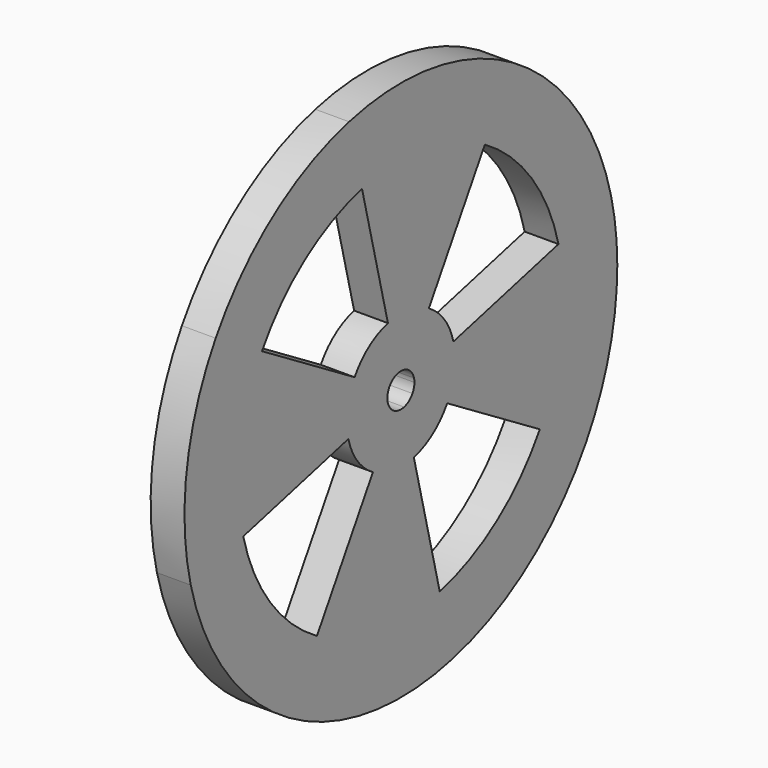
from build123d import *

# Parameters (mm, degrees)
F1_DEPTH = 3.175


with BuildPart() as f1:
    # F0 (on Right) → F1 (new body)
    with BuildSketch(Plane.YZ):
        with BuildLine():
            Line((-40.4511333859, 29.1073653109), (-36.3753204967, 26.6437996954))
            ThreePointArc((-36.3753204967, 26.6437996954), (-35.6929146046, 28.2235683845), (-35.4597376823, 29.9285538495))
            ThreePointArc((-35.4597376823, 29.9285538495), (-35.506060347, 30.6941595257), (-35.6443525017, 31.4485951564))
            Line((-35.6443525017, 31.4485951564), (-40.2683913872, 30.3085641762))
            ThreePointArc((-40.2683913872, 30.3085641762), (-40.2338183485, 30.1199552685), (-40.2222376823, 29.9285538495))
            ThreePointArc((-40.2222376823, 29.9285538495), (-40.2805319129, 29.5023074832), (-40.4511333859, 29.1073653109))
        make_face()
        with BuildLine():
            ThreePointArc((-40.2896963754, 23.7631686688), (-38.0460118676, 24.8141752957), (-36.3753204967, 26.6437996954))
            Line((-36.3753204967, 26.6437996954), (-40.4511333859, 29.1073653109))
            ThreePointArc((-40.4511333859, 29.1073653109), (-40.8688062286, 28.649959211), (-41.4297273556, 28.3872075543))
            Line((-41.4297273556, 28.3872075543), (-40.2896963754, 23.7631686688))
        make_face()
        with BuildLine():
            ThreePointArc((-35.4597376823, 29.9285538495), (-35.6929146046, 28.2235683845), (-36.3753204967, 26.6437996954))
            Line((-36.3753204967, 26.6437996954), (-25.5064861254, 20.0742913873))
            ThreePointArc((-25.5064861254, 20.0742913873), (-23.4592684491, 24.8135974547), (-22.7597376823, 29.9285538495))
            ThreePointArc((-22.7597376823, 29.9285538495), (-22.8987056762, 32.2253708783), (-23.3135821405, 34.4886777702))
            Line((-23.3135821405, 34.4886777702), (-35.6443525017, 31.4485951564))
            ThreePointArc((-35.6443525017, 31.4485951564), (-35.506060347, 30.6941595257), (-35.4597376823, 29.9285538495))
        make_face()
        with BuildLine():
            Line((-37.2496137616, 11.4323983076), (-40.2896963754, 23.7631686688))
            ThreePointArc((-40.2896963754, 23.7631686688), (-42.7647933931, 23.6507860464), (-45.0944918364, 24.4941366638))
            Line((-45.0944918364, 24.4941366638), (-51.6640001445, 13.6253022926))
            ThreePointArc((-51.6640001445, 13.6253022926), (-44.6749048146, 11.0952504402), (-37.2496137616, 11.4323983076))
        make_face()
        with BuildLine():
            ThreePointArc((-45.0944918364, 24.4941366638), (-42.7647933931, 23.6507860464), (-40.2896963754, 23.7631686688))
            Line((-40.2896963754, 23.7631686688), (-41.4297273556, 28.3872075543))
            ThreePointArc((-41.4297273556, 28.3872075543), (-42.04850161, 28.3591118987), (-42.6309262209, 28.5699495531))
            Line((-42.6309262209, 28.5699495531), (-45.0944918364, 24.4941366638))
        make_face()
        with BuildLine():
            ThreePointArc((-22.7597376823, 29.9285538495), (-23.4592684491, 24.8135974547), (-25.5064861254, 20.0742913873))
            Line((-25.5064861254, 20.0742913873), (-20.0720689398, 16.7895372333))
            ThreePointArc((-20.0720689398, 16.7895372333), (-17.3424453714, 23.1086119897), (-16.4097376823, 29.9285538495))
            ThreePointArc((-16.4097376823, 29.9285538495), (-16.5950283409, 32.9909765546), (-17.1481969599, 36.0087190771))
            Line((-17.1481969599, 36.0087190771), (-23.3135821405, 34.4886777702))
            ThreePointArc((-23.3135821405, 34.4886777702), (-22.8987056762, 32.2253708783), (-22.7597376823, 29.9285538495))
        make_face()
        with BuildLine():
            Line((-20.0720689398, 16.7895372333), (-25.5064861254, 20.0742913873))
            ThreePointArc((-25.5064861254, 20.0742913873), (-30.518560238, 14.5854181882), (-37.2496137616, 11.4323983076))
            Line((-37.2496137616, 11.4323983076), (-35.7295724547, 5.267013127))
            ThreePointArc((-35.7295724547, 5.267013127), (-26.7548344232, 9.4710396345), (-20.0720689398, 16.7895372333))
        make_face()
        with BuildLine():
            Line((-40.2683913872, 30.3085641762), (-35.6443525017, 31.4485951564))
            ThreePointArc((-35.6443525017, 31.4485951564), (-36.6953591286, 33.6922796642), (-38.5249835283, 35.3629710351))
            Line((-38.5249835283, 35.3629710351), (-40.9885491438, 31.2871581459))
            ThreePointArc((-40.9885491438, 31.2871581459), (-40.5311430439, 30.8694853032), (-40.2683913872, 30.3085641762))
        make_face()
        with BuildLine():
            ThreePointArc((-47.975122863, 28.4085125426), (-46.9241162361, 26.1648280347), (-45.0944918364, 24.4941366638))
            Line((-45.0944918364, 24.4941366638), (-42.6309262209, 28.5699495531))
            ThreePointArc((-42.6309262209, 28.5699495531), (-43.0883323208, 28.9876223958), (-43.3510839775, 29.5485435227))
            Line((-43.3510839775, 29.5485435227), (-47.975122863, 28.4085125426))
        make_face()
        with BuildLine():
            Line((-35.7295724547, 5.267013127), (-37.2496137616, 11.4323983076))
            ThreePointArc((-37.2496137616, 11.4323983076), (-44.6749048146, 11.0952504402), (-51.6640001445, 13.6253022926))
            Line((-51.6640001445, 13.6253022926), (-54.9487542985, 8.1908851069))
            ThreePointArc((-54.9487542985, 8.1908851069), (-45.6299605253, 4.8174826371), (-35.7295724547, 5.267013127))
        make_face()
        with BuildLine():
            Line((-40.9885491438, 31.2871581459), (-38.5249835283, 35.3629710351))
            ThreePointArc((-38.5249835283, 35.3629710351), (-40.8546819716, 36.2063216525), (-43.3297789892, 36.0939390301))
            Line((-43.3297789892, 36.0939390301), (-42.1897480091, 31.4699001446))
            ThreePointArc((-42.1897480091, 31.4699001446), (-41.5709737547, 31.4979958002), (-40.9885491438, 31.2871581459))
        make_face()
        with BuildLine():
            ThreePointArc((-43.3297789892, 36.0939390301), (-40.8546819716, 36.2063216525), (-38.5249835283, 35.3629710351))
            Line((-38.5249835283, 35.3629710351), (-31.9554752202, 46.2318054064))
            ThreePointArc((-31.9554752202, 46.2318054064), (-38.9445705501, 48.7618572587), (-46.3698616031, 48.4247093913))
            Line((-46.3698616031, 48.4247093913), (-43.3297789892, 36.0939390301))
        make_face()
        with BuildLine():
            ThreePointArc((-31.9554752202, 46.2318054064), (-26.4666020211, 41.2197312938), (-23.3135821405, 34.4886777702))
            Line((-23.3135821405, 34.4886777702), (-17.1481969599, 36.0087190771))
            ThreePointArc((-17.1481969599, 36.0087190771), (-21.3522234673, 44.9834571086), (-28.6707210662, 51.666222592))
            Line((-28.6707210662, 51.666222592), (-31.9554752202, 46.2318054064))
        make_face()
        with BuildLine():
            Line((-60.3058932242, 25.3684299287), (-47.975122863, 28.4085125426))
            ThreePointArc((-47.975122863, 28.4085125426), (-48.0875054854, 30.8836095602), (-47.244154868, 33.2133080035))
            Line((-47.244154868, 33.2133080035), (-58.1129892392, 39.7828163116))
            ThreePointArc((-58.1129892392, 39.7828163116), (-60.6430410916, 32.7937209817), (-60.3058932242, 25.3684299287))
        make_face()
        with BuildLine():
            ThreePointArc((-47.244154868, 33.2133080035), (-48.0875054854, 30.8836095602), (-47.975122863, 28.4085125426))
            Line((-47.975122863, 28.4085125426), (-43.3510839775, 29.5485435227))
            ThreePointArc((-43.3510839775, 29.5485435227), (-43.3791796331, 30.1673177771), (-43.1683419788, 30.749742388))
            Line((-43.1683419788, 30.749742388), (-47.244154868, 33.2133080035))
        make_face()
        with BuildLine():
            Line((-54.9487542985, 8.1908851069), (-51.6640001445, 13.6253022926))
            ThreePointArc((-51.6640001445, 13.6253022926), (-57.1528733436, 18.6373764051), (-60.3058932242, 25.3684299287))
            Line((-60.3058932242, 25.3684299287), (-66.4712784048, 23.8483886218))
            ThreePointArc((-66.4712784048, 23.8483886218), (-62.2672518974, 14.8736505903), (-54.9487542985, 8.1908851069))
        make_face()
        with BuildLine():
            Line((-47.244154868, 33.2133080035), (-43.1683419788, 30.749742388))
            ThreePointArc((-43.1683419788, 30.749742388), (-42.750669136, 31.2071484879), (-42.1897480091, 31.4699001446))
            Line((-42.1897480091, 31.4699001446), (-43.3297789892, 36.0939390301))
            ThreePointArc((-43.3297789892, 36.0939390301), (-45.5734634971, 35.0429324032), (-47.244154868, 33.2133080035))
        make_face()
        with BuildLine():
            ThreePointArc((-46.3698616031, 48.4247093913), (-38.9445705501, 48.7618572587), (-31.9554752202, 46.2318054064))
            Line((-31.9554752202, 46.2318054064), (-28.6707210662, 51.666222592))
            ThreePointArc((-28.6707210662, 51.666222592), (-37.9895148394, 55.0396250618), (-47.88990291, 54.5900945719))
            Line((-47.88990291, 54.5900945719), (-46.3698616031, 48.4247093913))
        make_face()
        with BuildLine():
            Line((-66.4712784048, 23.8483886218), (-60.3058932242, 25.3684299287))
            ThreePointArc((-60.3058932242, 25.3684299287), (-60.6430410916, 32.7937209817), (-58.1129892392, 39.7828163116))
            Line((-58.1129892392, 39.7828163116), (-63.5474064249, 43.0675704656))
            ThreePointArc((-63.5474064249, 43.0675704656), (-66.9208088947, 33.7487766925), (-66.4712784048, 23.8483886218))
        make_face()
        with BuildLine():
            ThreePointArc((-58.1129892392, 39.7828163116), (-53.1009151267, 45.2716895107), (-46.3698616031, 48.4247093913))
            Line((-46.3698616031, 48.4247093913), (-47.88990291, 54.5900945719))
            ThreePointArc((-47.88990291, 54.5900945719), (-56.8646409415, 50.3860680645), (-63.5474064249, 43.0675704656))
            Line((-63.5474064249, 43.0675704656), (-58.1129892392, 39.7828163116))
        make_face()
    extrude(amount=F1_DEPTH)


solid = f1.part
